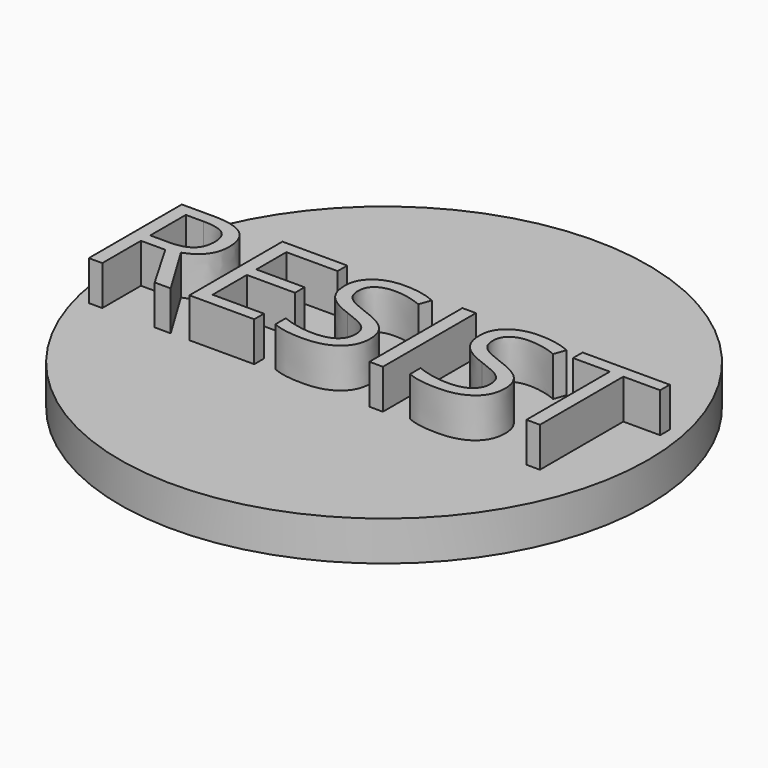
from build123d import *

# Parameters (mm, degrees)
F0_R         = 10
F1_DEPTH     = 1.5
F2_TEXT_SIZE = 6.1695882427
F3_DEPTH     = 1.5


# Not quite as in the source:
# - Text() gives the source's letters only with a copy of the font that has no kerning and outlines rounded to 1/6400 em; it was checked with that copy


with BuildPart() as f1:
    # F0 (on Top) → F1 (new body)
    with BuildSketch(Plane.XY):
        Circle(F0_R)
    extrude(amount=F1_DEPTH)

    # F2 (on face) → F3 (join)
    with BuildSketch(Plane.XY.offset(1.5)):
        with Locations((-9.8063700442, -2.4837607263)):
            Text('RESIST', F2_TEXT_SIZE, font='Open Sans', text_align=(TextAlign.LEFT, TextAlign.BOTTOM))
    extrude(amount=F3_DEPTH)


solid = f1.part
